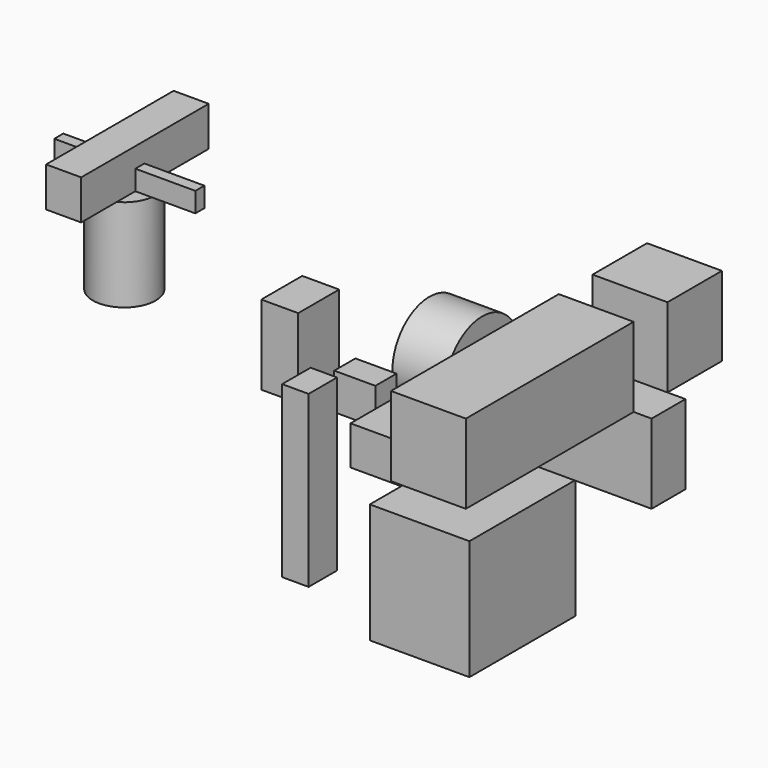
from build123d import *

# Parameters (mm, degrees)
F0_W      = 78.9292352274
F0_H      = 70.1791113243
F1_DEPTH  = 50.8
F2_W      = 96.850451082
F2_H      = 74.6815614402
F3_DEPTH  = 127
F4_W      = 70.7993283868
F4_H      = 98.2494205236
F5_DEPTH  = 152.4
F6_W      = 68.2949870825
F6_H      = 326.1379003525
F7_DEPTH  = 50.8
F8_R      = 88.7062581377
F9_DEPTH  = 101.6
F10_W     = 317.314684391
F10_H     = 81.1350904405
F11_DEPTH = 152.4
F12_W     = 191.2417113781
F12_H     = 229.7623949125
F13_DEPTH = 254
F14_R     = 60.1952157033
F15_DEPTH = 177.8
F17_DEPTH = 38.1
F18_W     = 67.3751235008
F18_H     = 176.0733984411
F19_DEPTH = 76.2
F20_W     = 143.7404751778
F20_H     = 130.599565804
F21_DEPTH = 152.4
F20_H_2   = 402.5698415935


# Not quite as in the source:
# - a feature names something its author has since deleted; it is built from what else it names


with BuildPart() as f1:
    # F0 (on Front) → F1 (new body)
    with BuildSketch(Plane.XZ):
        with Locations((-26.0592526756, 22.2907965071)):
            Rectangle(F0_W, F0_H)
    extrude(amount=F1_DEPTH)


with BuildPart() as f3:
    # F2 (on Front) → F3 (new body)
    with BuildSketch(Plane.XZ):
        with Locations((75.0986728817, -8.023692295)):
            Rectangle(F2_W, F2_H)
    extrude(amount=F3_DEPTH)


with BuildPart() as f5:
    # F4 (on Top) → F5 (new body)
    with BuildSketch(Plane.XY):
        with Locations((-145.6297449768, -32.2464182973)):
            Rectangle(F4_W, F4_H)
    extrude(amount=F5_DEPTH)


with BuildPart() as f7:
    # F6 (on Right) → F7 (new body)
    with BuildSketch(Plane.YZ):
        with Locations((-223.5160246491, -23.0616927147)):
            Rectangle(F6_W, F6_H)
    extrude(amount=F7_DEPTH)


with BuildPart() as f9:
    # F8 (on Right) → F9 (new body)
    with BuildSketch(Plane.YZ):
        with Locations((95.4723358154, 55.3811565042)):
            Circle(F8_R)
    extrude(amount=F9_DEPTH)


with BuildPart() as f11:
    # F10 (on Top) → F11 (new body)
    with BuildSketch(Plane.XY):
        with Locations((358.4956228733, 22.8078756481)):
            Rectangle(F10_W, F10_H)
    extrude(amount=F11_DEPTH)


with BuildPart() as f13:
    # F12 (on Front) → F13 (new body)
    with BuildSketch(Plane.XZ):
        with Locations((260.9308212996, -125.8234879933)):
            Rectangle(F12_W, F12_H)
    extrude(amount=F13_DEPTH)


with BuildPart() as f15:
    # F14 (on Top) → F15 (new body)
    with BuildSketch(Plane.XY):
        with Locations((-545.6547141075, 45.6993207335)):
            Circle(F14_R)
    extrude(amount=F15_DEPTH)

    # F16 (on face) → F17 (join)
    with BuildSketch(Plane.XY.offset(177.8)):
        with BuildLine():
            Line((-604.4325111577, 58.6852580309), (-673.0360388756, 58.6852580309))
            Line((-673.0360388756, 58.6852580309), (-673.0360388756, 37.0256043971))
            Line((-673.0360388756, 37.0256043971), (-605.221740544, 37.0256043971))
            ThreePointArc((-605.221740544, 37.0256043971), (-605.810008641, 47.8912452669), (-604.4325111577, 58.6852580309))
        make_face()
        with BuildLine():
            Line((-486.8769170573, 58.6852580309), (-604.4325111577, 58.6852580309))
            ThreePointArc((-604.4325111577, 58.6852580309), (-605.810008641, 47.8912452669), (-605.221740544, 37.0256043971))
            Line((-605.221740544, 37.0256043971), (-486.087687671, 37.0256043971))
            ThreePointArc((-486.087687671, 37.0256043971), (-485.6167511228, 41.3511033735), (-485.4594984042, 45.6993207335))
            ThreePointArc((-485.4594984042, 45.6993207335), (-485.814902253, 52.230852773), (-486.8769170573, 58.6852580309))
        make_face()
        with BuildLine():
            Line((-402.3371636868, 58.6852580309), (-486.8769170573, 58.6852580309))
            ThreePointArc((-486.8769170573, 58.6852580309), (-485.814902253, 52.230852773), (-485.4594984042, 45.6993207335))
            ThreePointArc((-485.4594984042, 45.6993207335), (-485.6167511228, 41.3511033735), (-486.087687671, 37.0256043971))
            Line((-486.087687671, 37.0256043971), (-402.3371636868, 37.0256043971))
            Line((-402.3371636868, 37.0256043971), (-402.3371636868, 58.6852580309))
        make_face()
    extrude(amount=F17_DEPTH)

    # F18 (on face) → F19 (join)
    with BuildSketch(Plane.XY.offset(177.8)):
        with BuildLine():
            Line((-584.9188566208, -92.848777771), (-517.54373312, -92.848777771))
            Line((-517.54373312, -92.848777771), (-517.54373312, -7.5288366785))
            ThreePointArc((-517.54373312, -7.5288366785), (-552.4033425041, -14.1163963342), (-584.9188566208, 0.0726716536))
            Line((-584.9188566208, 0.0726716536), (-584.9188566208, -92.848777771))
        make_face()
        with BuildLine():
            ThreePointArc((-584.9188566208, 0.0726716536), (-552.4033425041, -14.1163963342), (-517.54373312, -7.5288366785))
            Line((-517.54373312, -7.5288366785), (-517.54373312, 37.0256043971))
            Line((-517.54373312, 37.0256043971), (-584.9188566208, 37.0256043971))
            Line((-584.9188566208, 37.0256043971), (-584.9188566208, 0.0726716536))
        make_face()
        with Locations((-551.2312948704, 125.0623036176)):
            Rectangle(F18_W, F18_H)
    extrude(amount=F19_DEPTH)


with BuildPart() as f21:
    # F20 (on face) → F21 (new body)
    with BuildSketch(Plane.XY.offset(152.4)):
        with Locations((410.8542501926, 128.6752037704)):
            Rectangle(F20_W, F20_H)
    extrude(amount=F21_DEPTH)


with BuildPart() as f21b:
    # F20 (on face) → F21, piece 2 (new body)
    with BuildSketch(Plane.XY.offset(152.4)):
        with Locations((410.8542501926, -219.0445903689)):
            Rectangle(F20_W, F20_H_2)
    extrude(amount=F21_DEPTH)


solid = Compound([f1.part, f3.part, f5.part, f7.part, f9.part, f11.part, f13.part, f15.part, f21.part, f21b.part])
